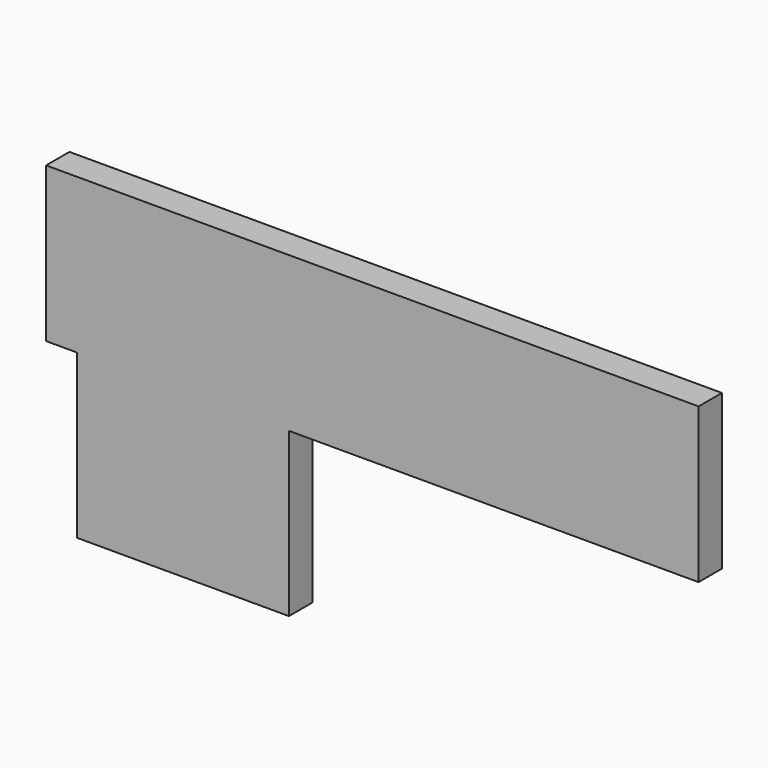
from build123d import *

# Parameters (mm, degrees)
F9_W      = 8.9488632511
F9_H      = 47.4289786071
F10_DEPTH = 100
F11_W     = 65
F11_H     = 8.9488632511
F12_DEPTH = 50


# Not quite as in the source:
# - a feature of the source that left no trace in its solid (it failed there, or was rolled back) is left out
# - the program builds the solid bodies; features that only make, move or delete a surface that nothing else refers to are left out


with BuildPart() as f10:
    # F9 (on Right) → F10 (new body, symmetric)
    with BuildSketch(Plane.YZ):
        with Locations((1.2304667616, 7.4946740642)):
            Rectangle(F9_W, F9_H)
    extrude(amount=F10_DEPTH, both=True)

    # F11 (on face) → F12 (join)
    with BuildSketch(Plane(origin=(0, 0, -16.2198152393), x_dir=(1, 0, 0), z_dir=(0, 0, -1))):
        with Locations((-58.0593782663, -1.2304667616)):
            Rectangle(F11_W, F11_H)
    extrude(amount=F12_DEPTH)


solid = f10.part
